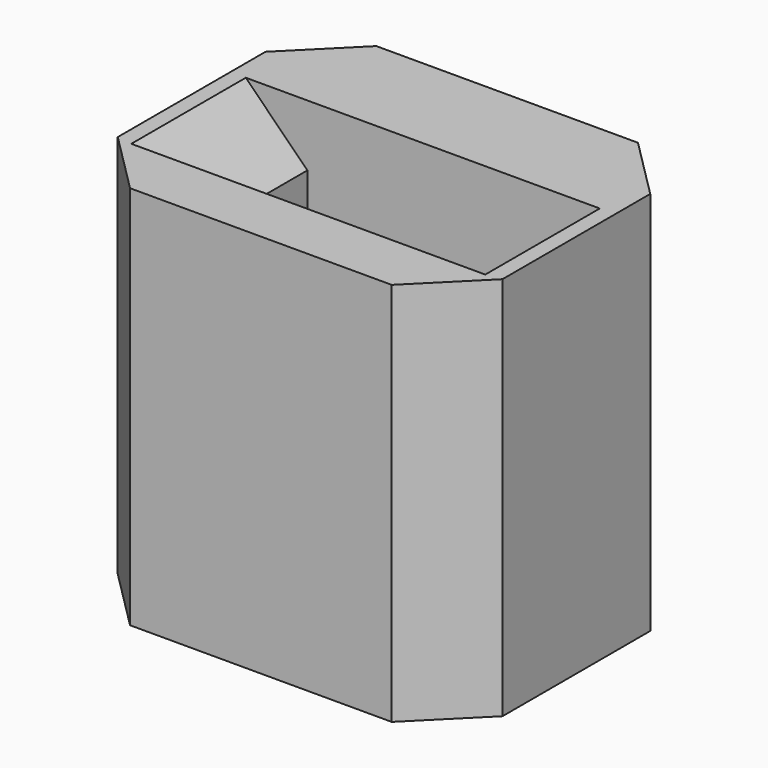
from build123d import *

# Parameters (mm, degrees)
F0_W         = 25
F0_H         = 20
F0_W_2       = 15
F0_H_2       = 6.3
F1_DEPTH     = 25
F2_W         = 15
F2_H         = 6.3
F3_DEPTH     = 2
F4_SIZE      = 4
F5_SIZE      = 3
F6_T1_DEPTH  = 15
F6_T6_DEPTH  = 6.1776695297
F6_T11_DEPTH = 6.1776695297


# Not quite as in the source:
# - a fillet or chamfer that OpenCascade refuses, or shapes differently, is made with other operations: its cross-section is extruded or revolved along the edge and cut away or added


with BuildPart() as f1:
    # F0 (on Top) → F1 (new body)
    with BuildSketch(Plane.XY):
        Rectangle(F0_W, F0_H)
        Rectangle(F0_W_2, F0_H_2, mode=Mode.SUBTRACT)
    extrude(amount=F1_DEPTH)

    # F2 (on face) → F3 (join)
    with BuildSketch(Plane(origin=(0, 0, 0), x_dir=(1, 0, 0), z_dir=(0, 0, -1))):
        Rectangle(F2_W, F2_H)
    extrude(amount=-F3_DEPTH)

    # F4
    f4_edges = [f1.edges().sort_by_distance(p)[0] for p in [
        (-7.5, 0, 25),
        (7.5, 0, 25),
        (-12.5, -10, 12.5),
        (12.5, -10, 12.5),
        (12.5, 10, 12.5),
        (-12.5, 10, 12.5),
    ]]
    chamfer(f4_edges, length=F4_SIZE)

    # F5
    f5_edges = [f1.edges().sort_by_distance(p)[0] for p in [
        (0, -3.15, 25),
    ]]
    chamfer(f5_edges, length=F5_SIZE)

    # F6: fillet of radius 5 on 1 edges, made by hand

    # F6_s2 → F6_t1 (cut)
    with BuildSketch(Plane.YZ.offset(-7.5)):
        with BuildLine():
            ThreePointArc((-4.6144660941, 23.4644660941), (-3.5306023374, 21.84234935), (-3.15, 19.9289321881))
            Line((-3.15, 19.9289321881), (-3.15, 22))
            Line((-3.15, 22), (-4.6144660941, 23.4644660941))
        make_face()
    extrude(amount=F6_T1_DEPTH, mode=Mode.SUBTRACT)


with BuildPart() as f6_tool4:
    # F6_s5 → F6_t6 (new body)
    with BuildSketch(Plane.YZ.offset(13.6776695297)):
        with BuildLine():
            ThreePointArc((-4.6144660941, 23.4644660941), (-3.5306023374, 21.84234935), (-3.15, 19.9289321881))
            Line((-3.15, 19.9289321881), (-3.15, 22))
            Line((-3.15, 22), (-4.6144660941, 23.4644660941))
        make_face()
    extrude(amount=-F6_T6_DEPTH)

    split(bisect_by=Plane(origin=(-6.75, 0, 6.75), x_dir=(0, 1, 0), z_dir=(-0.7071067812, 0, 0.7071067812)), keep=Keep.TOP)


with BuildPart() as f1_1:
    add(f1.part)

    # F6_t3: cut F6_tool4
    add(f6_tool4.part, mode=Mode.SUBTRACT)


with BuildPart() as f6_tool9:
    # F6_s10 → F6_t11 (new body)
    with BuildSketch(Plane.YZ.offset(-7.5)):
        with BuildLine():
            ThreePointArc((-4.6144660941, 23.4644660941), (-3.5306023374, 21.84234935), (-3.15, 19.9289321881))
            Line((-3.15, 19.9289321881), (-3.15, 22))
            Line((-3.15, 22), (-4.6144660941, 23.4644660941))
        make_face()
    extrude(amount=-F6_T11_DEPTH)

    split(bisect_by=Plane(origin=(6.75, 0, 6.75), x_dir=(0, 1, 0), z_dir=(0.7071067812, 0, 0.7071067812)), keep=Keep.TOP)


with BuildPart() as f1_2:
    add(f1_1.part)

    # F6_t8: cut F6_tool9
    add(f6_tool9.part, mode=Mode.SUBTRACT)


solid = f1_2.part
